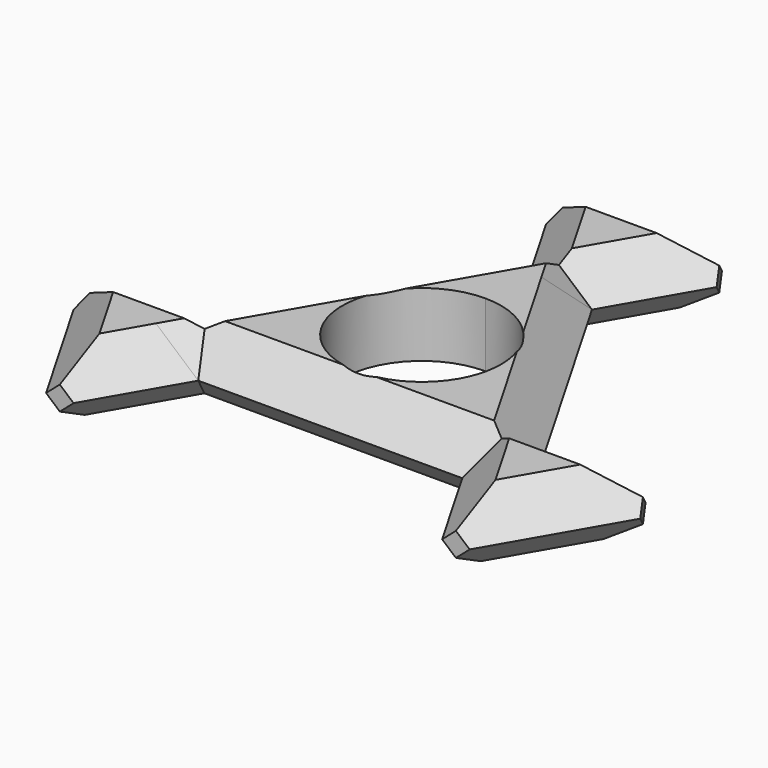
from build123d import *

# Parameters (mm, degrees)
F1_DEPTH      = 8.89
F2_DEPTH      = 8.89
F3_SIZE       = 3.81
F4_SIZE       = 3.81
F5_T1_DEPTH   = 45.9464028027
F5_T3_DEPTH   = 45.9464028027
F5_T5_DEPTH   = 45.9464028027
F5_T10_DEPTH  = 40.6103682544
F5_T15_DEPTH  = 40.6103682544
F5_T20_DEPTH  = 62.7124373511
F5_T26_DEPTH  = 62.7124373511
F5_T32_DEPTH  = 40.6103682544
F5_T37_DEPTH  = 40.6103682544
F5_T42_DEPTH  = 62.7124373511
F5_T48_DEPTH  = 40.6103682544
F5_T53_DEPTH  = 40.6103682544
F5_T58_DEPTH  = 29.9382991577
F5_T63_DEPTH  = 29.9382991577
F5_T68_DEPTH  = 29.9382991577
F5_T73_DEPTH  = 29.9382991577
F5_T78_DEPTH  = 29.9382991577
F5_T83_DEPTH  = 29.9382991577
F5_T88_DEPTH  = 29.9382991577
F5_T93_DEPTH  = 29.9382991577
F5_T98_DEPTH  = 29.9382991577
F5_T103_DEPTH = 29.9382991577
F5_T108_DEPTH = 29.9382991577
F5_T113_DEPTH = 29.9382991577


# Not quite as in the source:
# - a fillet or chamfer that OpenCascade refuses, or shapes differently, is made with other operations: its cross-section is extruded or revolved along the edge and cut away or added


with BuildPart() as f1:
    # F0 (on Top) → F1 (new body)
    with BuildSketch(Plane.XY):
        with BuildLine():
            ThreePointArc((0, 11), (7.7781745931, 7.7781745931), (11, 0))
            ThreePointArc((11, 0), (10.6251840892, -2.8470094961), (9.5262794416, -5.5))
            Line((9.5262794416, -5.5), (13.7190518225, -7.9206982628))
            Line((13.7190518225, -7.9206982628), (22.8650863708, -7.9206982628))
            Line((22.8650863708, -7.9206982628), (4.5730172742, 23.7620947883))
            Line((4.5730172742, 23.7620947883), (0, 15.8413965255))
            Line((0, 15.8413965255), (0, 11))
        make_face()
        with BuildLine():
            Line((13.7190518225, -7.9206982628), (9.5262794416, -5.5))
            ThreePointArc((9.5262794416, -5.5), (0, -11), (-9.5262794416, -5.5))
            Line((-9.5262794416, -5.5), (-13.7190518225, -7.9206982628))
            Line((-13.7190518225, -7.9206982628), (-18.2920690967, -15.8413965255))
            Line((-18.2920690967, -15.8413965255), (18.2920690967, -15.8413965255))
            Line((18.2920690967, -15.8413965255), (13.7190518225, -7.9206982628))
        make_face()
        with BuildLine():
            ThreePointArc((-9.5262794416, -5.5), (-9.5262794416, 5.5), (0, 11))
            Line((0, 11), (0, 15.8413965255))
            Line((0, 15.8413965255), (-4.5730172742, 23.7620947883))
            Line((-4.5730172742, 23.7620947883), (-22.8650863708, -7.9206982628))
            Line((-22.8650863708, -7.9206982628), (-13.7190518225, -7.9206982628))
            Line((-13.7190518225, -7.9206982628), (-9.5262794416, -5.5))
        make_face()
    extrude(amount=F1_DEPTH)

    # F0 (on Top) → F2 (join)
    with BuildSketch(Plane.XY):
        with BuildLine():
            ThreePointArc((0, 11), (7.7781745931, 7.7781745931), (11, 0))
            ThreePointArc((11, 0), (10.6251840892, -2.8470094961), (9.5262794416, -5.5))
            Line((9.5262794416, -5.5), (13.7190518225, -7.9206982628))
            Line((13.7190518225, -7.9206982628), (22.8650863708, -7.9206982628))
            Line((22.8650863708, -7.9206982628), (4.5730172742, 23.7620947883))
            Line((4.5730172742, 23.7620947883), (0, 15.8413965255))
            Line((0, 15.8413965255), (0, 11))
        make_face()
        with BuildLine():
            ThreePointArc((-9.5262794416, -5.5), (-9.5262794416, 5.5), (0, 11))
            Line((0, 11), (0, 15.8413965255))
            Line((0, 15.8413965255), (-4.5730172742, 23.7620947883))
            Line((-4.5730172742, 23.7620947883), (-22.8650863708, -7.9206982628))
            Line((-22.8650863708, -7.9206982628), (-13.7190518225, -7.9206982628))
            Line((-13.7190518225, -7.9206982628), (-9.5262794416, -5.5))
        make_face()
        with BuildLine():
            Line((13.7190518225, -7.9206982628), (9.5262794416, -5.5))
            ThreePointArc((9.5262794416, -5.5), (0, -11), (-9.5262794416, -5.5))
            Line((-9.5262794416, -5.5), (-13.7190518225, -7.9206982628))
            Line((-13.7190518225, -7.9206982628), (-18.2920690967, -15.8413965255))
            Line((-18.2920690967, -15.8413965255), (18.2920690967, -15.8413965255))
            Line((18.2920690967, -15.8413965255), (13.7190518225, -7.9206982628))
        make_face()
        Polygon((-4.5730172742, 23.7620947883), (0, 15.8413965255), (0, 31.682793051), align=None)
        Polygon((0, 31.682793051), (0, 15.8413965255), (4.5730172742, 23.7620947883), align=None)
        Polygon((22.8650863708, -7.9206982628), (13.7190518225, -7.9206982628), (27.438103645, -15.8413965255), align=None)
        Polygon((27.438103645, -15.8413965255), (13.7190518225, -7.9206982628), (18.2920690967, -15.8413965255), align=None)
        Polygon((-18.2920690967, -15.8413965255), (-13.7190518225, -7.9206982628), (-27.438103645, -15.8413965255), align=None)
        Polygon((-27.438103645, -15.8413965255), (-13.7190518225, -7.9206982628), (-22.8650863708, -7.9206982628), align=None)
        Polygon((-4.5730172742, 23.7620947883), (0, 31.682793051), (4.5730172742, 23.7620947883), (13.7190518225, 39.6034913138), (-13.7190518225, 39.6034913138), align=None)
        Polygon((22.8650863708, -7.9206982628), (27.438103645, -15.8413965255), (18.2920690967, -15.8413965255), (27.438103645, -31.682793051), (41.1571554675, -7.9206982628), align=None)
        Polygon((-18.2920690967, -15.8413965255), (-27.438103645, -15.8413965255), (-22.8650863708, -7.9206982628), (-41.1571554675, -7.9206982628), (-27.438103645, -31.682793051), align=None)
    extrude(amount=F2_DEPTH)

    # F3
    f3_edges = [f1.edges().sort_by_distance(p)[0] for p in [
        (-22.865086, -23.762095, 0),
        (-34.29763, -19.801746, 0),
        (-32.011121, -7.920698, 0),
        (0, -15.841397, 0),
        (-13.719052, 7.920698, 0),
        (-9.146035, 31.682793, 0),
        (9.146035, 31.682793, 0),
        (13.719052, 7.920698, 0),
        (32.011121, -7.920698, 0),
        (34.29763, -19.801746, 0),
        (22.865086, -23.762095, 0),
        (0, 39.603491, 0),
    ]]
    chamfer(f3_edges, length=F3_SIZE)

    # F4
    f4_edges = [f1.edges().sort_by_distance(p)[0] for p in [
        (27.438104, -31.682793, 6.35),
        (41.157155, -7.920698, 6.35),
        (13.719052, 39.603491, 6.35),
        (-27.438104, -31.682793, 6.35),
        (-13.719052, 39.603491, 6.35),
        (-41.157155, -7.920698, 6.35),
    ]]
    chamfer(f4_edges, length=F4_SIZE)

    # F5: chamfer of 5.08 on 18 edges, made by hand

    # F5_s2 → F5_t1 (cut)
    with BuildSketch(Plane.YZ.offset(-22.9732014014)):
        Polygon((34.5234913138, 8.89), (39.6034913138, 3.81), (39.6034913138, 8.89), align=None)
    extrude(amount=F5_T1_DEPTH, mode=Mode.SUBTRACT)

    # F5_s4 → F5_t3 (cut)
    with BuildSketch(Plane(origin=(-11.4866007007, -19.8953760198, 0), x_dir=(0, 0, 1), z_dir=(0.5, 0.8660254038, 0))):
        Polygon((8.89, 34.5234913138), (3.81, 39.6034913138), (8.89, 39.6034913138), align=None)
    extrude(amount=F5_T3_DEPTH, mode=Mode.SUBTRACT)

    # F5_s6 → F5_t5 (cut)
    with BuildSketch(Plane(origin=(-11.4866007007, 19.8953760198, 0), x_dir=(0, 0, 1), z_dir=(0.5, -0.8660254038, 0))):
        Polygon((8.89, 34.5234913138), (3.81, 39.6034913138), (8.89, 39.6034913138), align=None)
    extrude(amount=F5_T5_DEPTH, mode=Mode.SUBTRACT)


with BuildPart() as f5_tool8:
    # F5_s9 → F5_t10 (new body)
    with BuildSketch(Plane(origin=(4.900468396, 8.4878602427, 0), x_dir=(0, 0, 1), z_dir=(0.5, 0.8660254038, 0))):
        Polygon((8.89, -13.0006982628), (3.81, -7.9206982628), (8.89, -7.9206982628), align=None)
    extrude(amount=F5_T10_DEPTH)

    split(bisect_by=Plane(origin=(8.5093043055, 4.9128491314, 9.8256982628), x_dir=(-0.5, 0.8660254038, 0), z_dir=(0.6123724357, 0.3535533906, 0.7071067812)), keep=Keep.TOP)


with BuildPart() as f1_1:
    add(f1.part)

    # F5_t7: cut F5_tool8
    add(f5_tool8.part, mode=Mode.SUBTRACT)


with BuildPart() as f5_tool13:
    # F5_s14 → F5_t15 (new body)
    with BuildSketch(Plane(origin=(-25.2056525232, 43.6574708081, 0), x_dir=(0, 0, 1), z_dir=(0.5, -0.8660254038, 0))):
        Polygon((8.89, -13.0006982628), (3.81, -7.9206982628), (8.89, -7.9206982628), align=None)
    extrude(amount=F5_T15_DEPTH)

    split(bisect_by=Plane(origin=(-8.5093043055, 4.9128491314, 9.8256982628), x_dir=(-0.5, -0.8660254038, 0), z_dir=(-0.6123724357, 0.3535533906, 0.7071067812)), keep=Keep.TOP)


with BuildPart() as f1_2:
    add(f1_1.part)

    # F5_t12: cut F5_tool13
    add(f5_tool13.part, mode=Mode.SUBTRACT)


with BuildPart() as f5_tool18:
    # F5_s19 → F5_t20 (new body)
    with BuildSketch(Plane(origin=(15.6781093378, 27.1552819396, 0), x_dir=(0, 0, 1), z_dir=(-0.5, -0.8660254038, 0))):
        Polygon((8.89, 10.7613965255), (3.81, 15.8413965255), (8.89, 15.8413965255), align=None)
    extrude(amount=F5_T20_DEPTH)

    split(bisect_by=Plane(origin=(1.7799845614, 1.0276745657, -2.0553491314), x_dir=(0.5, -0.8660254038, 0), z_dir=(-0.6123724357, -0.3535533906, 0.7071067812)), keep=Keep.TOP)

    split(bisect_by=Plane(origin=(0, -2.0553491314, -2.0553491314), x_dir=(1, 0, 0), z_dir=(0, 0.7071067812, 0.7071067812)), keep=Keep.TOP)


with BuildPart() as f1_3:
    add(f1_2.part)

    # F5_t17: cut F5_tool18
    add(f5_tool18.part, mode=Mode.SUBTRACT)


with BuildPart() as f5_tool24:
    # F5_s25 → F5_t26 (new body)
    with BuildSketch(Plane(origin=(15.6781093378, -27.1552819396, 0), x_dir=(0, 0, 1), z_dir=(-0.5, 0.8660254038, 0))):
        Polygon((8.89, 10.7613965255), (3.81, 15.8413965255), (8.89, 15.8413965255), align=None)
    extrude(amount=F5_T26_DEPTH)

    split(bisect_by=Plane(origin=(0, -2.0553491314, -2.0553491314), x_dir=(1, 0, 0), z_dir=(0, 0.7071067812, 0.7071067812)), keep=Keep.TOP)

    split(bisect_by=Plane(origin=(-1.7799845614, 1.0276745657, -2.0553491314), x_dir=(0.5, 0.8660254038, 0), z_dir=(0.6123724357, -0.3535533906, 0.7071067812)), keep=Keep.TOP)


with BuildPart() as f1_4:
    add(f1_3.part)

    # F5_t23: cut F5_tool24
    add(f5_tool24.part, mode=Mode.SUBTRACT)


with BuildPart() as f5_tool30:
    # F5_s31 → F5_t32 (new body)
    with BuildSketch(Plane.YZ.offset(50.4113050464)):
        Polygon((-13.0006982628, 8.89), (-7.9206982628, 3.81), (-7.9206982628, 8.89), align=None)
    extrude(amount=-F5_T32_DEPTH)

    split(bisect_by=Plane(origin=(8.5093043055, 4.9128491314, 9.8256982628), x_dir=(-0.5, 0.8660254038, 0), z_dir=(0.6123724357, 0.3535533906, 0.7071067812)), keep=Keep.TOP)


with BuildPart() as f1_5:
    add(f1_4.part)

    # F5_t29: cut F5_tool30
    add(f5_tool30.part, mode=Mode.SUBTRACT)


with BuildPart() as f5_tool35:
    # F5_s36 → F5_t37 (new body)
    with BuildSketch(Plane(origin=(4.900468396, -8.4878602427, 0), x_dir=(0, 0, 1), z_dir=(0.5, -0.8660254038, 0))):
        Polygon((8.89, -13.0006982628), (3.81, -7.9206982628), (8.89, -7.9206982628), align=None)
    extrude(amount=F5_T37_DEPTH)

    split(bisect_by=Plane(origin=(0, -9.8256982628, 9.8256982628), x_dir=(1, 0, 0), z_dir=(0, -0.7071067812, 0.7071067812)), keep=Keep.TOP)


with BuildPart() as f1_6:
    add(f1_5.part)

    # F5_t34: cut F5_tool35
    add(f5_tool35.part, mode=Mode.SUBTRACT)


with BuildPart() as f5_tool40:
    # F5_s41 → F5_t42 (new body)
    with BuildSketch(Plane.YZ.offset(-31.3562186755)):
        Polygon((-15.8413965255, 3.81), (-10.7613965255, 8.89), (-15.8413965255, 8.89), align=None)
    extrude(amount=F5_T42_DEPTH)

    split(bisect_by=Plane(origin=(-1.7799845614, 1.0276745657, -2.0553491314), x_dir=(0.5, 0.8660254038, 0), z_dir=(0.6123724357, -0.3535533906, 0.7071067812)), keep=Keep.TOP)

    split(bisect_by=Plane(origin=(1.7799845614, 1.0276745657, -2.0553491314), x_dir=(0.5, -0.8660254038, 0), z_dir=(-0.6123724357, -0.3535533906, 0.7071067812)), keep=Keep.TOP)


with BuildPart() as f1_7:
    add(f1_6.part)

    # F5_t39: cut F5_tool40
    add(f5_tool40.part, mode=Mode.SUBTRACT)


with BuildPart() as f5_tool46:
    # F5_s47 → F5_t48 (new body)
    with BuildSketch(Plane(origin=(-25.2056525232, -43.6574708081, 0), x_dir=(0, 0, 1), z_dir=(0.5, 0.8660254038, 0))):
        Polygon((3.81, -7.9206982628), (8.89, -13.0006982628), (8.89, -7.9206982628), align=None)
    extrude(amount=F5_T48_DEPTH)

    split(bisect_by=Plane(origin=(0, -9.8256982628, 9.8256982628), x_dir=(1, 0, 0), z_dir=(0, -0.7071067812, 0.7071067812)), keep=Keep.TOP)


with BuildPart() as f1_8:
    add(f1_7.part)

    # F5_t45: cut F5_tool46
    add(f5_tool46.part, mode=Mode.SUBTRACT)


with BuildPart() as f5_tool51:
    # F5_s52 → F5_t53 (new body)
    with BuildSketch(Plane.YZ.offset(-9.800936792)):
        Polygon((-13.0006982628, 8.89), (-7.9206982628, 3.81), (-7.9206982628, 8.89), align=None)
    extrude(amount=-F5_T53_DEPTH)

    split(bisect_by=Plane(origin=(-8.5093043055, 4.9128491314, 9.8256982628), x_dir=(-0.5, -0.8660254038, 0), z_dir=(-0.6123724357, 0.3535533906, 0.7071067812)), keep=Keep.TOP)


with BuildPart() as f1_9:
    add(f1_8.part)

    # F5_t50: cut F5_tool51
    add(f5_tool51.part, mode=Mode.SUBTRACT)


with BuildPart() as f5_tool56:
    # F5_s57 → F5_t58 (new body)
    with BuildSketch(Plane(origin=(-21.2036266119, -36.7257585966, 0), x_dir=(0, 0, 1), z_dir=(0.5, 0.8660254038, 0))):
        Polygon((8.89, -23.3032362626), (3.81, -28.3832362626), (8.89, -28.3832362626), align=None)
    extrude(amount=F5_T58_DEPTH)

    split(bisect_by=Plane(origin=(-18.7985931723, -10.8533728284, 21.7067456569), x_dir=(0.5, -0.8660254038, 0), z_dir=(-0.6123724357, -0.3535533906, 0.7071067812)), keep=Keep.TOP)


with BuildPart() as f1_10:
    add(f1_9.part)

    # F5_t55: cut F5_tool56
    add(f5_tool56.part, mode=Mode.SUBTRACT)


with BuildPart() as f5_tool61:
    # F5_s62 → F5_t63 (new body)
    with BuildSketch(Plane(origin=(-21.2036266119, -36.7257585966, 0), x_dir=(0, 0, 1), z_dir=(0.5, 0.8660254038, 0))):
        Polygon((8.89, -23.3032362626), (3.81, -28.3832362626), (8.89, -28.3832362626), align=None)
    extrude(amount=F5_T63_DEPTH)

    split(bisect_by=Plane(origin=(0, -2.0553491314, -2.0553491314), x_dir=(1, 0, 0), z_dir=(0, 0.7071067812, 0.7071067812)), keep=Keep.TOP)


with BuildPart() as f1_11:
    add(f1_10.part)

    # F5_t60: cut F5_tool61
    add(f5_tool61.part, mode=Mode.SUBTRACT)


with BuildPart() as f5_tool66:
    # F5_s67 → F5_t68 (new body)
    with BuildSketch(Plane.YZ.offset(-12.4689540661)):
        Polygon((-28.3832362626, 3.81), (-23.3032362626, 8.89), (-28.3832362626, 8.89), align=None)
    extrude(amount=-F5_T68_DEPTH)

    split(bisect_by=Plane(origin=(-1.7799845614, 1.0276745657, -2.0553491314), x_dir=(0.5, 0.8660254038, 0), z_dir=(0.6123724357, -0.3535533906, 0.7071067812)), keep=Keep.TOP)


with BuildPart() as f1_12:
    add(f1_11.part)

    # F5_t65: cut F5_tool66
    add(f5_tool66.part, mode=Mode.SUBTRACT)


with BuildPart() as f5_tool71:
    # F5_s72 → F5_t73 (new body)
    with BuildSketch(Plane.YZ.offset(-12.4689540661)):
        Polygon((-28.3832362626, 3.81), (-23.3032362626, 8.89), (-28.3832362626, 8.89), align=None)
    extrude(amount=-F5_T73_DEPTH)

    split(bisect_by=Plane(origin=(-18.7985931723, -10.8533728284, 21.7067456569), x_dir=(0.5, -0.8660254038, 0), z_dir=(-0.6123724357, -0.3535533906, 0.7071067812)), keep=Keep.TOP)


with BuildPart() as f1_13:
    add(f1_12.part)

    # F5_t70: cut F5_tool71
    add(f5_tool71.part, mode=Mode.SUBTRACT)


with BuildPart() as f5_tool76:
    # F5_s77 → F5_t78 (new body)
    with BuildSketch(Plane.YZ.offset(12.4689540661)):
        Polygon((-23.3032362626, 8.89), (-28.3832362626, 3.81), (-28.3832362626, 8.89), align=None)
    extrude(amount=F5_T78_DEPTH)

    split(bisect_by=Plane(origin=(1.7799845614, 1.0276745657, -2.0553491314), x_dir=(0.5, -0.8660254038, 0), z_dir=(-0.6123724357, -0.3535533906, 0.7071067812)), keep=Keep.TOP)


with BuildPart() as f1_14:
    add(f1_13.part)

    # F5_t75: cut F5_tool76
    add(f5_tool76.part, mode=Mode.SUBTRACT)


with BuildPart() as f5_tool81:
    # F5_s82 → F5_t83 (new body)
    with BuildSketch(Plane.YZ.offset(12.4689540661)):
        Polygon((-23.3032362626, 8.89), (-28.3832362626, 3.81), (-28.3832362626, 8.89), align=None)
    extrude(amount=F5_T83_DEPTH)

    split(bisect_by=Plane(origin=(18.7985931723, -10.8533728284, 21.7067456569), x_dir=(0.5, 0.8660254038, 0), z_dir=(0.6123724357, -0.3535533906, 0.7071067812)), keep=Keep.TOP)


with BuildPart() as f1_15:
    add(f1_14.part)

    # F5_t80: cut F5_tool81
    add(f5_tool81.part, mode=Mode.SUBTRACT)


with BuildPart() as f5_tool86:
    # F5_s87 → F5_t88 (new body)
    with BuildSketch(Plane(origin=(21.2036266119, -36.7257585966, 0), x_dir=(0, 0, 1), z_dir=(-0.5, 0.8660254038, 0))):
        Polygon((8.89, 23.3032362626), (3.81, 28.3832362626), (8.89, 28.3832362626), align=None)
    extrude(amount=F5_T88_DEPTH)

    split(bisect_by=Plane(origin=(18.7985931723, -10.8533728284, 21.7067456569), x_dir=(0.5, 0.8660254038, 0), z_dir=(0.6123724357, -0.3535533906, 0.7071067812)), keep=Keep.TOP)


with BuildPart() as f1_16:
    add(f1_15.part)

    # F5_t85: cut F5_tool86
    add(f5_tool86.part, mode=Mode.SUBTRACT)


with BuildPart() as f5_tool91:
    # F5_s92 → F5_t93 (new body)
    with BuildSketch(Plane(origin=(21.2036266119, -36.7257585966, 0), x_dir=(0, 0, 1), z_dir=(-0.5, 0.8660254038, 0))):
        Polygon((8.89, 23.3032362626), (3.81, 28.3832362626), (8.89, 28.3832362626), align=None)
    extrude(amount=F5_T93_DEPTH)

    split(bisect_by=Plane(origin=(0, -2.0553491314, -2.0553491314), x_dir=(1, 0, 0), z_dir=(0, 0.7071067812, 0.7071067812)), keep=Keep.TOP)


with BuildPart() as f1_17:
    add(f1_16.part)

    # F5_t90: cut F5_tool91
    add(f5_tool91.part, mode=Mode.SUBTRACT)


with BuildPart() as f5_tool96:
    # F5_s97 → F5_t98 (new body)
    with BuildSketch(Plane(origin=(-6.2344770331, 10.7984309799, 0), x_dir=(0, 0, 1), z_dir=(-0.5, 0.8660254038, 0))):
        Polygon((8.89, 23.3032362626), (3.81, 28.3832362626), (8.89, 28.3832362626), align=None)
    extrude(amount=F5_T98_DEPTH)

    split(bisect_by=Plane(origin=(-1.7799845614, 1.0276745657, -2.0553491314), x_dir=(0.5, 0.8660254038, 0), z_dir=(0.6123724357, -0.3535533906, 0.7071067812)), keep=Keep.TOP)


with BuildPart() as f1_18:
    add(f1_17.part)

    # F5_t95: cut F5_tool96
    add(f5_tool96.part, mode=Mode.SUBTRACT)


with BuildPart() as f5_tool101:
    # F5_s102 → F5_t103 (new body)
    with BuildSketch(Plane(origin=(-6.2344770331, 10.7984309799, 0), x_dir=(0, 0, 1), z_dir=(-0.5, 0.8660254038, 0))):
        Polygon((8.89, 23.3032362626), (3.81, 28.3832362626), (8.89, 28.3832362626), align=None)
    extrude(amount=F5_T103_DEPTH)

    split(bisect_by=Plane(origin=(0, 21.7067456569, 21.7067456569), x_dir=(1, 0, 0), z_dir=(0, 0.7071067812, 0.7071067812)), keep=Keep.TOP)


with BuildPart() as f1_19:
    add(f1_18.part)

    # F5_t100: cut F5_tool101
    add(f5_tool101.part, mode=Mode.SUBTRACT)


with BuildPart() as f5_tool106:
    # F5_s107 → F5_t108 (new body)
    with BuildSketch(Plane(origin=(21.2036266119, 36.7257585966, 0), x_dir=(0, 0, 1), z_dir=(-0.5, -0.8660254038, 0))):
        Polygon((8.89, 23.3032362626), (3.81, 28.3832362626), (8.89, 28.3832362626), align=None)
    extrude(amount=F5_T108_DEPTH)

    split(bisect_by=Plane(origin=(0, 21.7067456569, 21.7067456569), x_dir=(1, 0, 0), z_dir=(0, 0.7071067812, 0.7071067812)), keep=Keep.TOP)


with BuildPart() as f1_20:
    add(f1_19.part)

    # F5_t105: cut F5_tool106
    add(f5_tool106.part, mode=Mode.SUBTRACT)


with BuildPart() as f5_tool111:
    # F5_s112 → F5_t113 (new body)
    with BuildSketch(Plane(origin=(21.2036266119, 36.7257585966, 0), x_dir=(0, 0, 1), z_dir=(-0.5, -0.8660254038, 0))):
        Polygon((8.89, 23.3032362626), (3.81, 28.3832362626), (8.89, 28.3832362626), align=None)
    extrude(amount=F5_T113_DEPTH)

    split(bisect_by=Plane(origin=(1.7799845614, 1.0276745657, -2.0553491314), x_dir=(0.5, -0.8660254038, 0), z_dir=(-0.6123724357, -0.3535533906, 0.7071067812)), keep=Keep.TOP)


with BuildPart() as f1_21:
    add(f1_20.part)

    # F5_t110: cut F5_tool111
    add(f5_tool111.part, mode=Mode.SUBTRACT)


solid = f1_21.part
